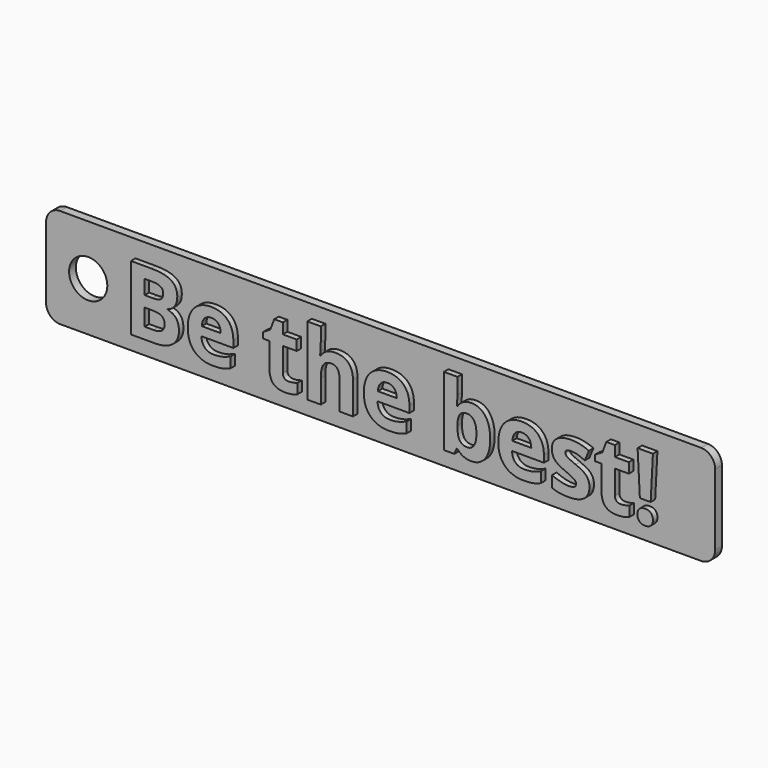
from build123d import *

# Parameters (mm, degrees)
F0_R         = 6.7639338093
F2_DEPTH     = 3
F1_TEXT_SIZE = 32.083623551
F3_DEPTH     = 5


# Not quite as in the source:
# - Text() gives the source's letters only with a copy of the font that has no kerning and outlines rounded to 1/6400 em; it was checked with that copy


with BuildPart() as f2:
    # F0 (on Front) → F2 (new body)
    with BuildSketch(Plane.XZ):
        with BuildLine():
            Line((166.3516062498, 37.0611285325), (-60.4029707611, 37.0611285325))
            ThreePointArc((-60.4029707611, 37.0611285325), (-63.938504667, 35.5966624384), (-65.4029707611, 32.0611285325))
            Line((-65.4029707611, 32.0611285325), (-65.4029707611, 6.8067655619))
            ThreePointArc((-65.4029707611, 6.8067655619), (-63.938504667, 3.271231656), (-60.4029707611, 1.8067655619))
            Line((-60.4029707611, 1.8067655619), (166.3516062498, 1.8067655619))
            ThreePointArc((166.3516062498, 1.8067655619), (169.8871401557, 3.271231656), (171.3516062498, 6.8067655619))
            Line((171.3516062498, 6.8067655619), (171.3516062498, 32.0611285325))
            ThreePointArc((171.3516062498, 32.0611285325), (169.8871401557, 35.5966624384), (166.3516062498, 37.0611285325))
        make_face()
        with Locations((-50.4989038408, 19.2050223704)):
            Circle(F0_R, mode=Mode.SUBTRACT)
    extrude(amount=F2_DEPTH)

    # F1 (on Front) → F3 (join)
    with BuildSketch(Plane.XZ):
        with Locations((-36.6634736474, 8.0732712522)):
            Text('Be the best!', F1_TEXT_SIZE, font='Open Sans', font_style=FontStyle.BOLD, text_align=(TextAlign.LEFT, TextAlign.BOTTOM))
    extrude(amount=F3_DEPTH)


solid = f2.part
